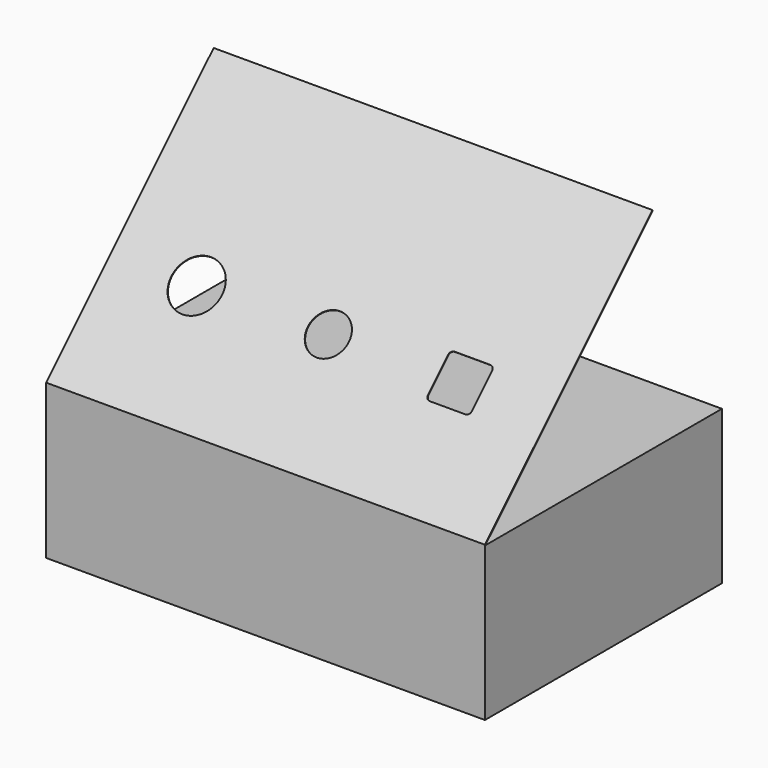
from build123d import *

# Parameters (mm, degrees)
F1_DEPTH = 127
F3_DEPTH = 0.4064


# Not quite as in the source:
# - the dataset's text gives a spline's control points without its knots; the knots are read off the source's solid


with BuildPart() as f1:
    # F0 (on Right) → F1 (new body, symmetric)
    with BuildSketch(Plane.YZ):
        Polygon((-171.45, 0), (0, 0), (0, 88.9), (-171.0436, 88.9), (-171.0436, 89.154), (-49.9291741697, 210.2684258303), (-50.2165423656, 210.5557940262), (-171.45, 89.3223363917), align=None)
    extrude(amount=F1_DEPTH, both=True)

    # F2 (on face) → F3 (cut, through all)
    with BuildSketch(Plane(origin=(0, -130.3861681959, 130.3861681959), x_dir=(1, 0, 0), z_dir=(0, -0.7071067812, 0.7071067812))):
        with BuildLine():
            add(Edge.make_bspline(
                [(87.2619638438, -4.1370739525), (87.7029332438, -3.6961045525), (87.9599304438, -3.0773605525), (87.9599304438, -2.4536127525)],
                knots=[1, 1, 1, 1, 2, 2, 2, 2], degree=3))
            Line((87.9599304438, -2.4536127525), (87.9599304438, 18.1838872475))
            add(Edge.make_bspline(
                [(87.9599304438, 18.1838872475), (87.9599304438, 18.8079652475), (87.7029332438, 19.4266838475), (87.2619638438, 19.8676532475)],
                knots=[0, 0, 0, 0, 1, 1, 1, 1], degree=3))
            add(Edge.make_bspline(
                [(87.2619638438, 19.8676532475), (86.8209944438, 20.3086480475), (86.2022504438, 20.5651372475), (85.5786804438, 20.5651372475)],
                knots=[1, 1, 1, 1, 2, 2, 2, 2], degree=3))
            Line((85.5786804438, 20.5651372475), (64.9411804438, 20.5651372475))
            add(Edge.make_bspline(
                [(64.9411804438, 20.5651372475), (64.3176104438, 20.5651372475), (63.6981806438, 20.3086480475), (63.2575668438, 19.8676532475)],
                knots=[0, 0, 0, 0, 1, 1, 1, 1], degree=3))
            add(Edge.make_bspline(
                [(63.2575668438, 19.8676532475), (62.8169276438, 19.4266838475), (62.5599304438, 18.8079652475), (62.5599304438, 18.1838872475)],
                knots=[1, 1, 1, 1, 2, 2, 2, 2], degree=3))
            Line((62.5599304438, 18.1838872475), (62.5599304438, -2.4536127525))
            add(Edge.make_bspline(
                [(62.5599304438, -2.4536127525), (62.5599304438, -3.0773605525), (62.8169276438, -3.6961045525), (63.2575668438, -4.1370739525)],
                knots=[0, 0, 0, 0, 1, 1, 1, 1], degree=3))
            add(Edge.make_bspline(
                [(63.2575668438, -4.1370739525), (63.6981806438, -4.5776877525), (64.3176104438, -4.8348627525), (64.9411804438, -4.8348627525)],
                knots=[1, 1, 1, 1, 2, 2, 2, 2], degree=3))
            Line((64.9411804438, -4.8348627525), (85.5786804438, -4.8348627525))
            add(Edge.make_bspline(
                [(85.5786804438, -4.8348627525), (86.2022504438, -4.8348627525), (86.8209944438, -4.5776877525), (87.2619638438, -4.1370739525)],
                knots=[0, 0, 0, 0, 1, 1, 1, 1], degree=3))
        make_face()
        with BuildLine():
            add(Edge.make_bspline(
                [(-66.7565495562, 18.2491652475), (-69.4747305562, 20.9673462475), (-73.2960081562, 22.5496646475), (-77.1400695562, 22.5496646475)],
                knots=[7, 7, 7, 7, 8, 8, 8, 8], degree=3))
            add(Edge.make_bspline(
                [(-77.1400695562, 22.5496646475), (-80.9841055562, 22.5496646475), (-84.8053831562, 20.9673462475), (-87.5235895562, 18.2491652475)],
                knots=[0, 0, 0, 0, 1, 1, 1, 1], degree=3))
            add(Edge.make_bspline(
                [(-87.5235895562, 18.2491652475), (-90.2424309562, 15.5306540475), (-91.8244445562, 11.7096812475), (-91.8244445562, 7.8651372475), (-91.8244445562, 4.0212790475), (-90.2424309562, 0.2003062475), (-87.5235895562, -2.5178747525)],
                knots=[1, 1, 1, 1, 2, 2, 2, 3, 3, 3, 3], degree=3))
            add(Edge.make_bspline(
                [(-87.5235895562, -2.5178747525), (-84.8053831562, -5.2367415525), (-80.9841055562, -6.8194155525), (-77.1400695562, -6.8194155525), (-73.2960081562, -6.8194155525), (-69.4747305562, -5.2367415525), (-66.7565495562, -2.5178747525)],
                knots=[3, 3, 3, 3, 4, 4, 4, 5, 5, 5, 5], degree=3))
            add(Edge.make_bspline(
                [(-66.7565495562, -2.5178747525), (-64.0383431562, 0.2003062475), (-62.4556945562, 4.0212790475), (-62.4556945562, 7.8651372475), (-62.4556945562, 11.7096812475), (-64.0383431562, 15.5306540475), (-66.7565495562, 18.2491652475)],
                knots=[5, 5, 5, 5, 6, 6, 6, 7, 7, 7, 7], degree=3))
        make_face()
        with BuildLine():
            add(Edge.make_bspline(
                [(7.4787096438, 16.2840688475), (5.2745484438, 18.4882554475), (2.1773994438, 19.7713872475), (-0.9397139562, 19.7713872475)],
                knots=[7, 7, 7, 7, 8, 8, 8, 8], degree=3))
            add(Edge.make_bspline(
                [(-0.9397139562, 19.7713872475), (-4.0572083562, 19.7713872475), (-7.1546621562, 18.4882554475), (-9.3588487562, 16.2840688475)],
                knots=[0, 0, 0, 0, 1, 1, 1, 1], degree=3))
            add(Edge.make_bspline(
                [(-9.3588487562, 16.2840688475), (-11.5630099562, 14.0799330475), (-12.8459639562, 10.9822506475), (-12.8459639562, 7.8651372475), (-12.8459639562, 4.7478206475), (-11.5630099562, 1.6501890475), (-9.3588487562, -0.5528037525)],
                knots=[1, 1, 1, 1, 2, 2, 2, 3, 3, 3, 3], degree=3))
            add(Edge.make_bspline(
                [(-9.3588487562, -0.5528037525), (-7.1546621562, -2.7569649525), (-4.0572083562, -4.0411127525), (-0.9397139562, -4.0411127525), (2.1773994438, -4.0411127525), (5.2745484438, -2.7569649525), (7.4787096438, -0.5528037525)],
                knots=[3, 3, 3, 3, 4, 4, 4, 5, 5, 5, 5], degree=3))
            add(Edge.make_bspline(
                [(7.4787096438, -0.5528037525), (9.6828962438, 1.6501890475), (10.9665360438, 4.7478206475), (10.9665360438, 7.8651372475), (10.9665360438, 10.9822506475), (9.6828962438, 14.0799330475), (7.4787096438, 16.2840688475)],
                knots=[5, 5, 5, 5, 6, 6, 6, 7, 7, 7, 7], degree=3))
        make_face()
    extrude(amount=-F3_DEPTH, mode=Mode.SUBTRACT)


solid = f1.part
